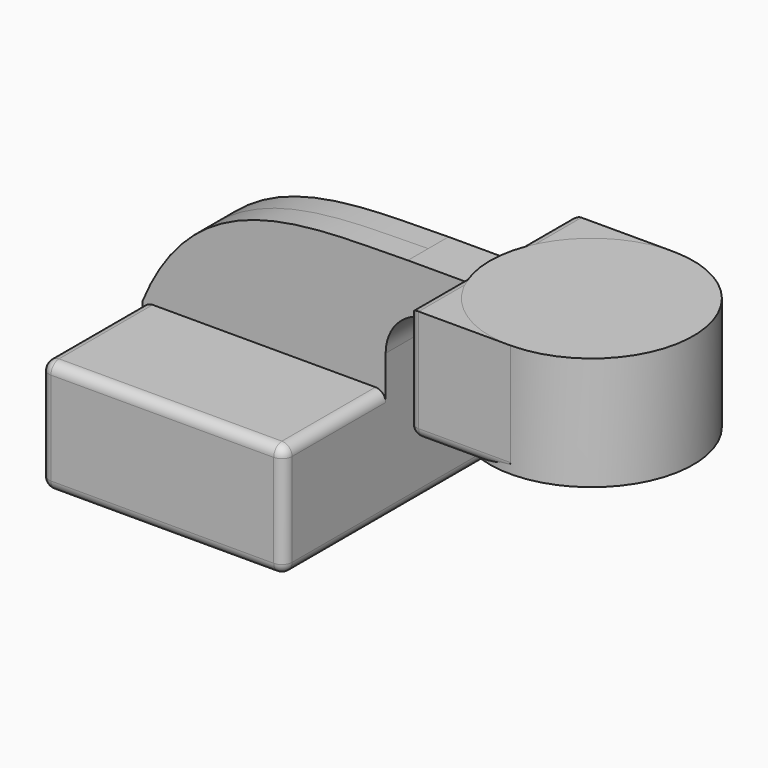
from build123d import *

# Parameters (mm, degrees)
F1_DEPTH     = 76.2
F2_DEPTH     = 12.7
F3_DEPTH     = 50.8
F4_T1_DEPTH  = 111.2565687561
F4_T3_DEPTH  = 46.5381988824
F4_T5_DEPTH  = 58.42
F4_T7_DEPTH  = 58.42
F4_T9_DEPTH  = 142.24
F4_T11_DEPTH = 127
F4_T13_DEPTH = 64.1849718046
F4_T15_DEPTH = 58.42
F4_T17_DEPTH = 91.44
F4_S21_W     = 5.1816
F4_S21_H     = 5.1816
F4_T22_DEPTH = 5.1816
F4_S27_W     = 5.1816
F4_S27_H     = 5.1816
F4_T28_DEPTH = 5.1816
F4_S33_W     = 5.1816
F4_S33_H     = 5.1816
F4_T34_DEPTH = 5.1816
F4_S39_W     = 5.1816
F4_S39_H     = 5.1816
F4_T40_DEPTH = 5.1816
F4_S45_W     = 5.1816
F4_S45_H     = 5.1816
F4_T46_DEPTH = 5.1816
F4_S51_W     = 5.1816
F4_S51_H     = 5.1816
F4_T52_DEPTH = 5.1816
F4_S57_W     = 5.1816
F4_S57_H     = 5.1816
F4_T58_DEPTH = 5.1816
F4_S63_W     = 5.1816
F4_S63_H     = 5.1816
F4_T64_DEPTH = 5.1816
F4_S69_W     = 5.1816
F4_S69_H     = 5.1816
F4_T70_DEPTH = 5.1816
F4_S75_W     = 5.1816
F4_S75_H     = 5.1816
F4_T76_DEPTH = 5.1816
F4_T82_DEPTH = 127
F4_T87_DEPTH = 127
F4_T92_DEPTH = 127


# Not quite as in the source:
# - a fillet or chamfer that OpenCascade refuses, or shapes differently, is made with other operations: its cross-section is extruded or revolved along the edge and cut away or added


with BuildPart() as f1:
    # F0 (on Front) → F1 (new body, symmetric)
    with BuildSketch(Plane.XZ):
        Polygon((-60.7082843781, -28.3490994412), (60.7082843781, -28.3490994412), (60.7082843781, 28.3490994412), (37.0862856507, 28.3490994412), (-60.7082843781, 28.3490994412), align=None)
    extrude(amount=F1_DEPTH, both=True)

    # F0 (on Front) → F2 (join, symmetric)
    with BuildSketch(Plane.XZ):
        with BuildLine():
            add(Edge.make_bspline(
                [(-60.7082843781, 28.3490994412), (-33.8972061735, 93.4263938061), (22.8176377988, 88.2478274848), (71.7955373972, 89.3411468321)],
                knots=[0, 0, 0, 0, 145.8673802807, 145.8673802807, 145.8673802807, 145.8673802807], degree=3))
            Line((-60.7082843781, 28.3490994412), (37.0862856507, 28.3490994412))
            Line((37.0862856507, 28.3490994412), (37.0862856507, 44.8936835745))
            ThreePointArc((37.0862856507, 44.8936835745), (46.7916042484, 73.0907984395), (71.7955373972, 89.3411468321))
        make_face()
        with BuildLine():
            Line((37.0862856507, 28.3490994412), (60.7082843781, 28.3490994412))
            Line((60.7082843781, 28.3490994412), (60.7082843781, 44.8936835745))
            ThreePointArc((60.7082843781, 44.8936835745), (64.6984303206, 57.5891124549), (75.2339748927, 65.7191481047))
            Line((75.2339748927, 65.7191481047), (102.6157526561, 65.7191481047))
            Line((102.6157526561, 65.7191481047), (102.6157526561, 89.3411468321))
            Line((102.6157526561, 89.3411468321), (71.7955373972, 89.3411468321))
            ThreePointArc((71.7955373972, 89.3411468321), (46.7916042484, 73.0907984395), (37.0862856507, 44.8936835745))
            Line((37.0862856507, 44.8936835745), (37.0862856507, 28.3490994412))
        make_face()
    extrude(amount=F2_DEPTH, both=True)

    # F0 (on Front) → F3 (join, symmetric)
    with BuildSketch(Plane.XZ):
        Polygon((102.6157526561, 94.0016340071), (102.6157526561, 89.3411468321), (102.6157526561, 65.7191481047), (102.6157526561, 37.4366622024), (153.4157526561, 37.4366622024), (153.4157526561, 94.0016340071), align=None)
    extrude(amount=F3_DEPTH, both=True)

    # F4: fillet of radius 5.08 on 21 edges, made by hand

    # F4_s2 → F4_t1 (cut)
    with BuildSketch(Plane.YZ.offset(-55.6282843781)):
        with BuildLine():
            ThreePointArc((71.12, 28.3490994412), (74.7121024484, 26.8612018896), (76.2, 23.2690994412))
            Line((76.2, 23.2690994412), (76.2, 28.3490994412))
            Line((76.2, 28.3490994412), (71.12, 28.3490994412))
        make_face()
        with BuildLine():
            ThreePointArc((71.12, -28.3490994412), (74.7121024484, -26.8612018896), (76.2, -23.2690994412))
            Line((76.2, -23.2690994412), (76.2, -28.3490994412))
            Line((76.2, -28.3490994412), (71.12, -28.3490994412))
        make_face()
        with BuildLine():
            ThreePointArc((-71.12, 28.3490994412), (-74.7121024484, 26.8612018896), (-76.2, 23.2690994412))
            Line((-76.2, 23.2690994412), (-76.2, 28.3490994412))
            Line((-76.2, 28.3490994412), (-71.12, 28.3490994412))
        make_face()
        with BuildLine():
            ThreePointArc((-71.12, -28.3490994412), (-74.7121024484, -26.8612018896), (-76.2, -23.2690994412))
            Line((-76.2, -23.2690994412), (-76.2, -28.3490994412))
            Line((-76.2, -28.3490994412), (-71.12, -28.3490994412))
        make_face()
    extrude(amount=F4_T1_DEPTH, mode=Mode.SUBTRACT)

    # F4_s4 → F4_t3 (cut)
    with BuildSketch(Plane.XY.offset(-23.2690994412)):
        with BuildLine():
            ThreePointArc((-60.7082843781, 71.12), (-59.2203868265, 74.7121024484), (-55.6282843781, 76.2))
            Line((-55.6282843781, 76.2), (-60.7082843781, 76.2))
            Line((-60.7082843781, 76.2), (-60.7082843781, 71.12))
        make_face()
        with BuildLine():
            ThreePointArc((60.7082843781, 71.12), (59.2203868265, 74.7121024484), (55.6282843781, 76.2))
            Line((55.6282843781, 76.2), (60.7082843781, 76.2))
            Line((60.7082843781, 76.2), (60.7082843781, 71.12))
        make_face()
        with BuildLine():
            ThreePointArc((60.7082843781, -71.12), (59.2203868265, -74.7121024484), (55.6282843781, -76.2))
            Line((55.6282843781, -76.2), (60.7082843781, -76.2))
            Line((60.7082843781, -76.2), (60.7082843781, -71.12))
        make_face()
        with BuildLine():
            ThreePointArc((-60.7082843781, -71.12), (-59.2203868265, -74.7121024484), (-55.6282843781, -76.2))
            Line((-55.6282843781, -76.2), (-60.7082843781, -76.2))
            Line((-60.7082843781, -76.2), (-60.7082843781, -71.12))
        make_face()
    extrude(amount=F4_T3_DEPTH, mode=Mode.SUBTRACT)

    # F4_s6 → F4_t5 (cut)
    with BuildSketch(Plane.XZ.offset(-71.12)):
        with BuildLine():
            ThreePointArc((-55.6282843781, 28.3490994412), (-59.2203868265, 26.8612018896), (-60.7082843781, 23.2690994412))
            Line((-60.7082843781, 23.2690994412), (-60.7082843781, 28.3490994412))
            Line((-60.7082843781, 28.3490994412), (-55.6282843781, 28.3490994412))
        make_face()
        with BuildLine():
            ThreePointArc((60.7082843781, 23.2690994412), (59.2203868265, 26.8612018896), (55.6282843781, 28.3490994412))
            Line((55.6282843781, 28.3490994412), (60.7082843781, 28.3490994412))
            Line((60.7082843781, 28.3490994412), (60.7082843781, 23.2690994412))
        make_face()
    extrude(amount=F4_T5_DEPTH, mode=Mode.SUBTRACT)

    # F4_s8 → F4_t7 (cut)
    with BuildSketch(Plane.XZ.offset(12.7)):
        with BuildLine():
            ThreePointArc((-55.6282843781, 28.3490994412), (-59.2203868265, 26.8612018896), (-60.7082843781, 23.2690994412))
            Line((-60.7082843781, 23.2690994412), (-60.7082843781, 28.3490994412))
            Line((-60.7082843781, 28.3490994412), (-55.6282843781, 28.3490994412))
        make_face()
        with BuildLine():
            ThreePointArc((60.7082843781, 23.2690994412), (59.2203868265, 26.8612018896), (55.6282843781, 28.3490994412))
            Line((55.6282843781, 28.3490994412), (60.7082843781, 28.3490994412))
            Line((60.7082843781, 28.3490994412), (60.7082843781, 23.2690994412))
        make_face()
    extrude(amount=F4_T7_DEPTH, mode=Mode.SUBTRACT)

    # F4_s10 → F4_t9 (cut)
    with BuildSketch(Plane.XZ.offset(-71.12)):
        with BuildLine():
            ThreePointArc((-60.7082843781, -23.2690994412), (-59.2203868265, -26.8612018896), (-55.6282843781, -28.3490994412))
            Line((-55.6282843781, -28.3490994412), (-60.7082843781, -28.3490994412))
            Line((-60.7082843781, -28.3490994412), (-60.7082843781, -23.2690994412))
        make_face()
        with BuildLine():
            ThreePointArc((60.7082843781, -23.2690994412), (59.2203868265, -26.8612018896), (55.6282843781, -28.3490994412))
            Line((55.6282843781, -28.3490994412), (60.7082843781, -28.3490994412))
            Line((60.7082843781, -28.3490994412), (60.7082843781, -23.2690994412))
        make_face()
    extrude(amount=F4_T9_DEPTH, mode=Mode.SUBTRACT)

    # F4_s12 → F4_t11 (cut)
    with BuildSketch(Plane.XZ.offset(-63.5)):
        with BuildLine():
            ThreePointArc((148.3357526561, 37.4366622024), (151.9278551045, 38.924559754), (153.4157526561, 42.5166622024))
            Line((153.4157526561, 42.5166622024), (153.4157526561, 37.4366622024))
            Line((153.4157526561, 37.4366622024), (148.3357526561, 37.4366622024))
        make_face()
    extrude(amount=F4_T11_DEPTH, mode=Mode.SUBTRACT)

    # F4_s14 → F4_t13 (cut)
    with BuildSketch(Plane.XY.offset(42.5166622024)):
        with BuildLine():
            ThreePointArc((102.6157526561, -45.72), (104.1036502077, -49.3121024484), (107.6957526561, -50.8))
            Line((107.6957526561, -50.8), (102.6157526561, -50.8))
            Line((102.6157526561, -50.8), (102.6157526561, -45.72))
        make_face()
        with BuildLine():
            ThreePointArc((102.6157526561, 45.72), (104.1036502077, 49.3121024484), (107.6957526561, 50.8))
            Line((107.6957526561, 50.8), (102.6157526561, 50.8))
            Line((102.6157526561, 50.8), (102.6157526561, 45.72))
        make_face()
    extrude(amount=F4_T13_DEPTH, mode=Mode.SUBTRACT)

    # F4_s16 → F4_t15 (cut)
    with BuildSketch(Plane.YZ.offset(107.6957526561)):
        with BuildLine():
            ThreePointArc((-45.72, 37.4366622024), (-49.3121024484, 38.924559754), (-50.8, 42.5166622024))
            Line((-50.8, 42.5166622024), (-50.8, 37.4366622024))
            Line((-50.8, 37.4366622024), (-45.72, 37.4366622024))
        make_face()
        with BuildLine():
            ThreePointArc((50.8, 42.5166622024), (49.3121024484, 38.924559754), (45.72, 37.4366622024))
            Line((45.72, 37.4366622024), (50.8, 37.4366622024))
            Line((50.8, 37.4366622024), (50.8, 42.5166622024))
        make_face()
    extrude(amount=F4_T15_DEPTH, mode=Mode.SUBTRACT)

    # F4_s18 → F4_t17 (cut)
    with BuildSketch(Plane.XZ.offset(-45.72)):
        with BuildLine():
            ThreePointArc((102.6157526561, 42.5166622024), (104.1036502077, 38.924559754), (107.6957526561, 37.4366622024))
            Line((107.6957526561, 37.4366622024), (102.6157526561, 37.4366622024))
            Line((102.6157526561, 37.4366622024), (102.6157526561, 42.5166622024))
        make_face()
    extrude(amount=F4_T17_DEPTH, mode=Mode.SUBTRACT)


with BuildPart() as f4_tool20:
    # F4_s21 → F4_t22 (new body)
    with BuildSketch(Plane.YZ.offset(-55.6282843781)):
        with Locations((73.7108, 25.8598994412)):
            Rectangle(F4_S21_W, F4_S21_H)
    extrude(amount=-F4_T22_DEPTH)

    # F4_s23 → F4_t24 (revolve, cut)
    with BuildSketch(Plane(origin=(-55.6282843781, 71.12, 23.2690994412), x_dir=(0, -0.7071067812, -0.7071067812), z_dir=(0, 0.7071067812, -0.7071067812))):
        with BuildLine():
            ThreePointArc((0, -5.08), (5.08, 0), (0, 5.08))
            Line((0, 5.08), (0, -5.08))
        make_face()
    revolve(axis=Axis((-55.6282843781, 71.12, 23.2690994412), (-1, 0, 0)), mode=Mode.SUBTRACT)


with BuildPart() as f1_1:
    add(f1.part)

    # F4_t19: cut F4_tool20
    add(f4_tool20.part, mode=Mode.SUBTRACT)


with BuildPart() as f4_tool26:
    # F4_s27 → F4_t28 (new body)
    with BuildSketch(Plane.XZ.offset(-71.12)):
        with Locations((58.2190843781, 25.8598994412)):
            Rectangle(F4_S27_W, F4_S27_H)
    extrude(amount=-F4_T28_DEPTH)

    # F4_s29 → F4_t30 (revolve, cut)
    with BuildSketch(Plane(origin=(55.6282843781, 71.12, 23.2690994412), x_dir=(-0.7071067812, 0, -0.7071067812), z_dir=(0.7071067812, 0, -0.7071067812))):
        with BuildLine():
            ThreePointArc((0, -5.08), (5.08, 0), (0, 5.08))
            Line((0, 5.08), (0, -5.08))
        make_face()
    revolve(axis=Axis((55.6282843781, 71.12, 23.2690994412), (0, 1, 0)), mode=Mode.SUBTRACT)


with BuildPart() as f1_2:
    add(f1_1.part)

    # F4_t25: cut F4_tool26
    add(f4_tool26.part, mode=Mode.SUBTRACT)


with BuildPart() as f4_tool32:
    # F4_s33 → F4_t34 (new body)
    with BuildSketch(Plane.YZ.offset(-55.6282843781)):
        with Locations((73.7108, -25.8598994412)):
            Rectangle(F4_S33_W, F4_S33_H)
    extrude(amount=-F4_T34_DEPTH)

    # F4_s35 → F4_t36 (revolve, cut)
    with BuildSketch(Plane(origin=(-55.6282843781, 71.12, -23.2690994412), x_dir=(0, -0.7071067812, 0.7071067812), z_dir=(0, -0.7071067812, -0.7071067812))):
        with BuildLine():
            ThreePointArc((0, -5.08), (5.08, 0), (0, 5.08))
            Line((0, 5.08), (0, -5.08))
        make_face()
    revolve(axis=Axis((-55.6282843781, 71.12, -23.2690994412), (-1, 0, 0)), mode=Mode.SUBTRACT)


with BuildPart() as f1_3:
    add(f1_2.part)

    # F4_t31: cut F4_tool32
    add(f4_tool32.part, mode=Mode.SUBTRACT)


with BuildPart() as f4_tool38:
    # F4_s39 → F4_t40 (new body)
    with BuildSketch(Plane.XY.offset(-23.2690994412)):
        with Locations((58.2190843781, 73.7108)):
            Rectangle(F4_S39_W, F4_S39_H)
    extrude(amount=-F4_T40_DEPTH)

    # F4_s41 → F4_t42 (revolve, cut)
    with BuildSketch(Plane(origin=(55.6282843781, 71.12, -23.2690994412), x_dir=(-0.7071067812, -0.7071067812, 0), z_dir=(0.7071067812, -0.7071067812, 0))):
        with BuildLine():
            ThreePointArc((0, -5.08), (5.08, 0), (0, 5.08))
            Line((0, 5.08), (0, -5.08))
        make_face()
    revolve(axis=Axis((55.6282843781, 71.12, -23.2690994412), (0, 0, -1)), mode=Mode.SUBTRACT)


with BuildPart() as f1_4:
    add(f1_3.part)

    # F4_t37: cut F4_tool38
    add(f4_tool38.part, mode=Mode.SUBTRACT)


with BuildPart() as f4_tool44:
    # F4_s45 → F4_t46 (new body)
    with BuildSketch(Plane.YZ.offset(-55.6282843781)):
        with Locations((-73.7108, 25.8598994412)):
            Rectangle(F4_S45_W, F4_S45_H)
    extrude(amount=-F4_T46_DEPTH)

    # F4_s47 → F4_t48 (revolve, cut)
    with BuildSketch(Plane(origin=(-55.6282843781, -71.12, 23.2690994412), x_dir=(0, 0.7071067812, -0.7071067812), z_dir=(0, 0.7071067812, 0.7071067812))):
        with BuildLine():
            ThreePointArc((0, -5.08), (5.08, 0), (0, 5.08))
            Line((0, 5.08), (0, -5.08))
        make_face()
    revolve(axis=Axis((-55.6282843781, -71.12, 23.2690994412), (-1, 0, 0)), mode=Mode.SUBTRACT)


with BuildPart() as f1_5:
    add(f1_4.part)

    # F4_t43: cut F4_tool44
    add(f4_tool44.part, mode=Mode.SUBTRACT)


with BuildPart() as f4_tool50:
    # F4_s51 → F4_t52 (new body)
    with BuildSketch(Plane.XZ.offset(71.12)):
        with Locations((58.2190843781, 25.8598994412)):
            Rectangle(F4_S51_W, F4_S51_H)
    extrude(amount=F4_T52_DEPTH)

    # F4_s53 → F4_t54 (revolve, cut)
    with BuildSketch(Plane(origin=(55.6282843781, -71.12, 23.2690994412), x_dir=(-0.7071067812, 0, -0.7071067812), z_dir=(-0.7071067812, 0, 0.7071067812))):
        with BuildLine():
            ThreePointArc((0, -5.08), (5.08, 0), (0, 5.08))
            Line((0, 5.08), (0, -5.08))
        make_face()
    revolve(axis=Axis((55.6282843781, -71.12, 23.2690994412), (0, -1, 0)), mode=Mode.SUBTRACT)


with BuildPart() as f1_6:
    add(f1_5.part)

    # F4_t49: cut F4_tool50
    add(f4_tool50.part, mode=Mode.SUBTRACT)


with BuildPart() as f4_tool56:
    # F4_s57 → F4_t58 (new body)
    with BuildSketch(Plane.YZ.offset(-55.6282843781)):
        with Locations((-73.7108, -25.8598994412)):
            Rectangle(F4_S57_W, F4_S57_H)
    extrude(amount=-F4_T58_DEPTH)

    # F4_s59 → F4_t60 (revolve, cut)
    with BuildSketch(Plane(origin=(-55.6282843781, -71.12, -23.2690994412), x_dir=(0, 0.7071067812, 0.7071067812), z_dir=(0, -0.7071067812, 0.7071067812))):
        with BuildLine():
            ThreePointArc((0, -5.08), (5.08, 0), (0, 5.08))
            Line((0, 5.08), (0, -5.08))
        make_face()
    revolve(axis=Axis((-55.6282843781, -71.12, -23.2690994412), (-1, 0, 0)), mode=Mode.SUBTRACT)


with BuildPart() as f1_7:
    add(f1_6.part)

    # F4_t55: cut F4_tool56
    add(f4_tool56.part, mode=Mode.SUBTRACT)


with BuildPart() as f4_tool62:
    # F4_s63 → F4_t64 (new body)
    with BuildSketch(Plane.XY.offset(-23.2690994412)):
        with Locations((58.2190843781, -73.7108)):
            Rectangle(F4_S63_W, F4_S63_H)
    extrude(amount=-F4_T64_DEPTH)

    # F4_s65 → F4_t66 (revolve, cut)
    with BuildSketch(Plane(origin=(55.6282843781, -71.12, -23.2690994412), x_dir=(-0.7071067812, 0.7071067812, 0), z_dir=(-0.7071067812, -0.7071067812, 0))):
        with BuildLine():
            ThreePointArc((0, -5.08), (5.08, 0), (0, 5.08))
            Line((0, 5.08), (0, -5.08))
        make_face()
    revolve(axis=Axis((55.6282843781, -71.12, -23.2690994412), (0, 0, -1)), mode=Mode.SUBTRACT)


with BuildPart() as f1_8:
    add(f1_7.part)

    # F4_t61: cut F4_tool62
    add(f4_tool62.part, mode=Mode.SUBTRACT)


with BuildPart() as f4_tool68:
    # F4_s69 → F4_t70 (new body)
    with BuildSketch(Plane.YZ.offset(107.6957526561)):
        with Locations((-48.3108, 39.9258622024)):
            Rectangle(F4_S69_W, F4_S69_H)
    extrude(amount=-F4_T70_DEPTH)

    # F4_s71 → F4_t72 (revolve, cut)
    with BuildSketch(Plane(origin=(107.6957526561, -45.72, 42.5166622024), x_dir=(0, 0.7071067812, 0.7071067812), z_dir=(0, -0.7071067812, 0.7071067812))):
        with BuildLine():
            ThreePointArc((0, -5.08), (5.08, 0), (0, 5.08))
            Line((0, 5.08), (0, -5.08))
        make_face()
    revolve(axis=Axis((107.6957526561, -45.72, 42.5166622024), (-1, 0, 0)), mode=Mode.SUBTRACT)


with BuildPart() as f1_9:
    add(f1_8.part)

    # F4_t67: cut F4_tool68
    add(f4_tool68.part, mode=Mode.SUBTRACT)


with BuildPart() as f4_tool74:
    # F4_s75 → F4_t76 (new body)
    with BuildSketch(Plane.YZ.offset(107.6957526561)):
        with Locations((48.3108, 39.9258622024)):
            Rectangle(F4_S75_W, F4_S75_H)
    extrude(amount=-F4_T76_DEPTH)

    # F4_s77 → F4_t78 (revolve, cut)
    with BuildSketch(Plane(origin=(107.6957526561, 45.72, 42.5166622024), x_dir=(0, -0.7071067812, 0.7071067812), z_dir=(0, -0.7071067812, -0.7071067812))):
        with BuildLine():
            ThreePointArc((0, -5.08), (5.08, 0), (0, 5.08))
            Line((0, 5.08), (0, -5.08))
        make_face()
    revolve(axis=Axis((107.6957526561, 45.72, 42.5166622024), (-1, 0, 0)), mode=Mode.SUBTRACT)


with BuildPart() as f1_10:
    add(f1_9.part)

    # F4_t73: cut F4_tool74
    add(f4_tool74.part, mode=Mode.SUBTRACT)


with BuildPart() as f4_tool80:
    # F4_s81 → F4_t82 (new body)
    with BuildSketch(Plane.XZ.offset(63.5)):
        with BuildLine():
            ThreePointArc((102.6157526561, 88.9216340071), (104.1036502077, 92.5137364555), (107.6957526561, 94.0016340071))
            Line((107.6957526561, 94.0016340071), (102.6157526561, 94.0016340071))
            Line((102.6157526561, 94.0016340071), (102.6157526561, 88.9216340071))
        make_face()
    extrude(amount=-F4_T82_DEPTH)

    split(bisect_by=Plane.XZ.offset(12.7), keep=Keep.TOP)


with BuildPart() as f1_11:
    add(f1_10.part)

    # F4_t79: cut F4_tool80
    add(f4_tool80.part, mode=Mode.SUBTRACT)


with BuildPart() as f4_tool85:
    # F4_s86 → F4_t87 (new body)
    with BuildSketch(Plane.XZ.offset(63.5)):
        with BuildLine():
            ThreePointArc((102.6157526561, 88.9216340071), (104.1036502077, 92.5137364555), (107.6957526561, 94.0016340071))
            Line((107.6957526561, 94.0016340071), (102.6157526561, 94.0016340071))
            Line((102.6157526561, 94.0016340071), (102.6157526561, 88.9216340071))
        make_face()
    extrude(amount=-F4_T87_DEPTH)

    split(bisect_by=Plane.XY.offset(89.3411468321), keep=Keep.TOP)


with BuildPart() as f1_12:
    add(f1_11.part)

    # F4_t84: cut F4_tool85
    add(f4_tool85.part, mode=Mode.SUBTRACT)


with BuildPart() as f4_tool90:
    # F4_s91 → F4_t92 (new body)
    with BuildSketch(Plane.XZ.offset(63.5)):
        with BuildLine():
            ThreePointArc((102.6157526561, 88.9216340071), (104.1036502077, 92.5137364555), (107.6957526561, 94.0016340071))
            Line((107.6957526561, 94.0016340071), (102.6157526561, 94.0016340071))
            Line((102.6157526561, 94.0016340071), (102.6157526561, 88.9216340071))
        make_face()
    extrude(amount=-F4_T92_DEPTH)

    split(bisect_by=Plane.XZ.offset(-12.7), keep=Keep.BOTTOM)


with BuildPart() as f1_13:
    add(f1_12.part)

    # F4_t89: cut F4_tool90
    add(f4_tool90.part, mode=Mode.SUBTRACT)


with BuildPart() as f5:
    # F0 (on Front) → F5 (revolve)
    with BuildSketch(Plane.XZ):
        Polygon((102.6157526561, 94.0016340071), (102.6157526561, 89.3411468321), (102.6157526561, 65.7191481047), (102.6157526561, 37.4366622024), (153.4157526561, 37.4366622024), (153.4157526561, 94.0016340071), align=None)
    revolve(axis=Axis((153.4157526561, 0, 65.7191481047), (0, 0, -1)))


solid = Compound([f1_13.part, f5.part])
